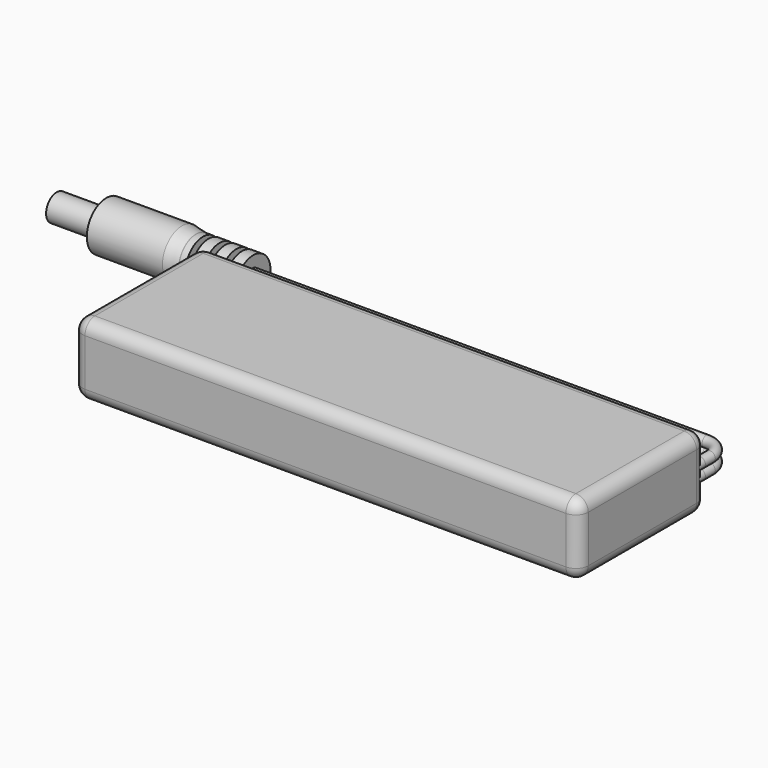
from build123d import *

# Parameters (mm, degrees)
F0_W         = 103.6193
F0_H         = 32.8168
F1_DEPTH     = 14.732
F2_R         = 2.54
F4_DEPTH     = 12.7
F4_FACE_R    = 1.0795
F12_R        = 4.445
F13_DEPTH    = 11.6713
F11_R        = 1.0795
F15_W        = 1.143
F15_H        = 2.0589674757
F15_H_2      = 3.7090053149
F16_DEPTH    = 24.13
F17_R        = 4.9911
F17_R_2      = 4.445
F18_DEPTH    = 18.415
F19_S5_R     = 4.445
F19_T6_DEPTH = 9
F21_R        = 2.72415
F22_DEPTH    = 1.27
F23_DEPTH    = 8.89
F24_R        = 1.0795
F25_DEPTH    = 8.89
F26_SIZE     = 0.635


# Not quite as in the source:
# - a fillet or chamfer that OpenCascade refuses, or shapes differently, is made with other operations: its cross-section is extruded or revolved along the edge and cut away or added


with BuildPart() as f1:
    # F0 (on Top) → F1 (new body)
    with BuildSketch(Plane.XY):
        with Locations((51.80965, -16.4084)):
            Rectangle(F0_W, F0_H)
    extrude(amount=F1_DEPTH)

    # F2
    f2_edges = [f1.edges().sort_by_distance(p)[0] for p in [
        (51.80965, -32.8168, 14.732),
        (51.80965, 0, 14.732),
        (0, -16.4084, 14.732),
        (103.6193, -16.4084, 14.732),
        (103.6193, -32.8168, 7.366),
        (103.6193, 0, 7.366),
        (103.6193, -16.4084, 0),
        (51.80965, 0, 0),
        (0, -16.4084, 0),
        (51.80965, -32.8168, 0),
        (0, 0, 7.366),
        (0, -32.8168, 7.366),
    ]]
    fillet(f2_edges, radius=F2_R)


with BuildPart() as f4:
    # F3 (on face) → F4 (new body)
    with BuildSketch(Plane(origin=(0, 0, 0), x_dir=(-1, 0, 0), z_dir=(0, 1, 0))):
        with BuildLine():
            ThreePointArc((-102.3098584272, 7.366), (-103.0731801975, 5.5231782297), (-101.2303584272, 6.2865))
            ThreePointArc((-101.2303584272, 6.2865), (-101.546536657, 7.0498217703), (-102.3098584272, 7.366))
        make_face()
    extrude(amount=-F4_DEPTH)

    # F9: sweep along a path in F7
    with BuildLine(Plane(origin=(0, 0, 6.2484), x_dir=(1, 0, 0), z_dir=(0, 0, -1))) as f9_path:
        Line((102.3098584272, 0), (102.3098584272, -2.54))
        ThreePointArc((102.3098584272, -2.54), (101.1939352636, -5.2340768363), (98.4998584272, -6.35))
        Line((98.4998584272, -6.35), (5.6628584272, -6.35))
    # F4_face (on face) → F9 (sweep)
    with BuildSketch(Plane(origin=(102.3098584272, 0, 6.2865), x_dir=(-1, 0, 0), z_dir=(0, 1, 0))):
        Circle(F4_FACE_R)
    sweep(path=f9_path.line)


with BuildPart() as f4b:
    # F3 (on face) → F4, piece 2 (new body)
    with BuildSketch(Plane(origin=(0, 0, 0), x_dir=(-1, 0, 0), z_dir=(0, 1, 0))):
        with BuildLine():
            ThreePointArc((-101.2303584272, 8.4455), (-103.0731801975, 9.2088217703), (-102.3098584272, 7.366))
            ThreePointArc((-102.3098584272, 7.366), (-101.546536657, 7.6821782297), (-101.2303584272, 8.4455))
        make_face()
    extrude(amount=-F4_DEPTH)

    # F10: sweep along a path in F8
    with BuildLine(Plane(origin=(0, 0, 8.4328), x_dir=(1, 0, 0), z_dir=(0, 0, -1))) as f10_path:
        Line((102.3098584272, 0), (102.3098584272, -2.54))
        ThreePointArc((102.3098584272, -2.54), (101.1939352636, -5.2340768363), (98.4998584272, -6.35))
        Line((98.4998584272, -6.35), (5.6628584272, -6.35))
    # F4_face (on face) → F10 (sweep)
    with BuildSketch(Plane(origin=(102.3098584272, 0, 6.2865), x_dir=(-1, 0, 0), z_dir=(0, 1, 0))):
        with Locations((0, 2.159)):
            Circle(F4_FACE_R)
    sweep(path=f10_path.line)

    # F12 (on face) → F13 (join)
    with BuildSketch(Plane(origin=(5.6628584272, 0, 0), x_dir=(0, -1, 0), z_dir=(-1, 0, 0))):
        with Locations((-6.35, 7.366)):
            Circle(F12_R)
        with BuildLine():
            ThreePointArc((-6.35, 7.366), (-5.5866782297, 7.0498217703), (-5.2705, 6.2865))
            ThreePointArc((-5.2705, 6.2865), (-7.1133217703, 5.5231782297), (-6.35, 7.366))
        make_face(mode=Mode.SUBTRACT)
        with BuildLine():
            ThreePointArc((-5.2705, 8.4455), (-5.5866782297, 7.6821782297), (-6.35, 7.366))
            ThreePointArc((-6.35, 7.366), (-7.1133217703, 9.2088217703), (-5.2705, 8.4455))
        make_face(mode=Mode.SUBTRACT)
        with BuildLine():
            ThreePointArc((-6.35, 7.366), (-7.1133217703, 5.5231782297), (-5.2705, 6.2865))
            ThreePointArc((-5.2705, 6.2865), (-5.5866782297, 7.0498217703), (-6.35, 7.366))
        make_face()
    extrude(amount=F13_DEPTH)

    # F11 (on face) → F13, piece 2 (join)
    with BuildSketch(Plane(origin=(5.6628584272, 0, 0), x_dir=(0, -1, 0), z_dir=(-1, 0, 0))):
        with Locations((-6.35, 8.4455)):
            Circle(F11_R)
    extrude(amount=F13_DEPTH)

    # F15 (on offset) → F16 (cut)
    with BuildSketch(Plane(origin=(0, 25.4, 0), x_dir=(-1, 0, 0), z_dir=(0, 1, 0))):
        with Locations((4.0526415728, 1.8915162622)):
            Rectangle(F15_W, F15_H)
        with Locations((4.0526415728, 4.7755026575)):
            Rectangle(F15_W, F15_H_2)
        with Locations((0.6236415728, 1.8915162622)):
            Rectangle(F15_W, F15_H)
        with Locations((0.6236415728, 4.7755026575)):
            Rectangle(F15_W, F15_H_2)
        with Locations((-2.8053584272, 1.8915162622)):
            Rectangle(F15_W, F15_H)
        with Locations((-2.8053584272, 4.7755026575)):
            Rectangle(F15_W, F15_H_2)
        with Locations((-2.8053584272, 9.9564973425)):
            Rectangle(F15_W, F15_H_2)
        with Locations((0.6236415728, 9.9564973425)):
            Rectangle(F15_W, F15_H_2)
        with Locations((-2.8053584272, 12.8404837378)):
            Rectangle(F15_W, F15_H)
        with Locations((0.6236415728, 12.8404837378)):
            Rectangle(F15_W, F15_H)
        with Locations((4.0526415728, 12.8404837378)):
            Rectangle(F15_W, F15_H)
        with Locations((4.0526415728, 9.9564973425)):
            Rectangle(F15_W, F15_H_2)
    extrude(amount=-F16_DEPTH, mode=Mode.SUBTRACT)

    # F17 (on face) → F18 (join)
    with BuildSketch(Plane(origin=(-6.0084415728, 0, 0), x_dir=(0, -1, 0), z_dir=(-1, 0, 0))):
        with Locations((-6.35, 7.366)):
            Circle(F17_R)
        with Locations((-6.35, 7.366)):
            Circle(F17_R_2, mode=Mode.SUBTRACT)
        with Locations((-6.35, 7.366)):
            Circle(F17_R_2)
    extrude(amount=F18_DEPTH)

    # F19: chamfer of 2.921 x 0.5588 on 1 edges, made by hand


with BuildPart() as f19_tool2:
    # F19_s3 → F19_t4 (revolve)
    with BuildSketch(Plane.XY.offset(7.366)):
        Polygon((-8.9294415728, 1.3589), (-6.0084415728, 1.9177), (-6.0084415728, 1.3589), align=None)
    revolve(axis=Axis((-6.0084415728, 6.35, 7.366), (-1, 0, 0)))

    # F19_s5 → F19_t6 (cut, symmetric)
    with BuildSketch(Plane.YZ.offset(-7.5)):
        with Locations((6.35, 7.366)):
            Circle(F19_S5_R)
    extrude(amount=F19_T6_DEPTH, both=True, mode=Mode.SUBTRACT)


with BuildPart() as f4b_1:
    add(f4b.part)

    # F19_t1: cut F19_tool2
    add(f19_tool2.part, mode=Mode.SUBTRACT)


with BuildPart() as f22:
    # F21 (on offset) → F22 (new body, through all)
    with BuildSketch(Plane(origin=(-25.6934415728, 0, 0), x_dir=(0, -1, 0), z_dir=(-1, 0, 0))):
        with Locations((-6.35, 7.366)):
            Circle(F21_R)
    extrude(amount=-F22_DEPTH)

    # F23 (add): a face of the model
    f23_faces = [f22.faces().sort_by_distance(p)[0] for p in [
        (-25.6934415728, 6.35, 7.366),
    ]]
    extrude(f23_faces, amount=F23_DEPTH)

    # F24 (on face) → F25 (cut, symmetric)
    with BuildSketch(Plane(origin=(-34.5834415728, 0, 0), x_dir=(0, -1, 0), z_dir=(-1, 0, 0))):
        with Locations((-6.35, 7.366)):
            Circle(F24_R)
    extrude(amount=F25_DEPTH, both=True, mode=Mode.SUBTRACT)

    # F26
    f26_edges = [f22.edges().sort_by_distance(p)[0] for p in [
        (-34.583442, 7.4295, 7.366),
    ]]
    chamfer(f26_edges, length=F26_SIZE)


solid = Compound([f1.part, f4.part, f4b_1.part, f22.part])
